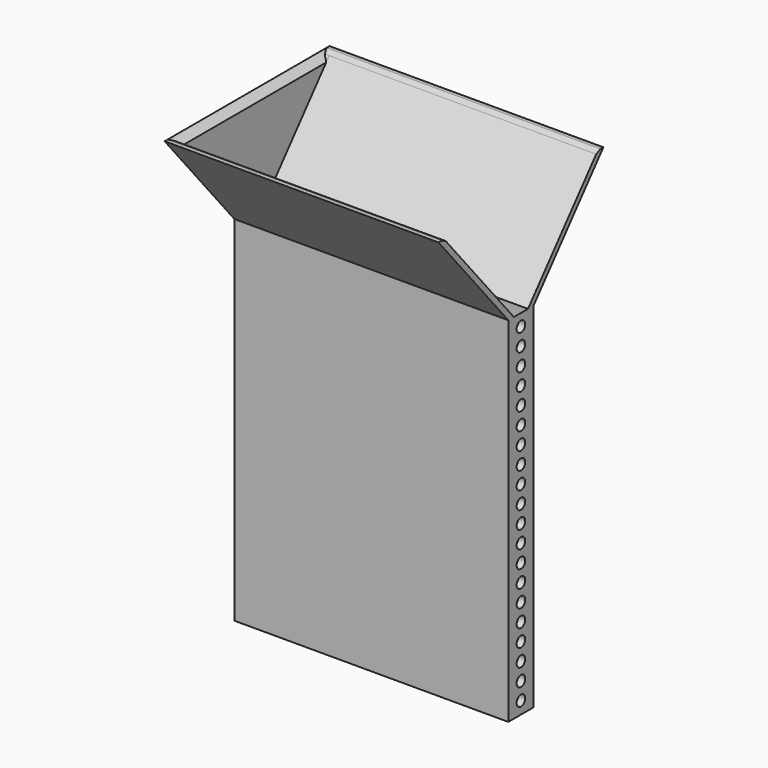
from build123d import *

# Parameters (mm, degrees)
F0_W         = 79
F0_H         = 9.1
F0_W_2       = 75
F0_H_2       = 5.1
F1_DEPTH     = 100
F0_W_3       = 55
F0_H_3       = 2.1
F2_DEPTH     = 2
F3_R         = 1.55
F4_DEPTH     = 79.001
F6_DEPTH     = 79
F7_DEPTH     = 2
F8_T1_DEPTH  = 5.1
F8_T3_DEPTH  = 79.5142210175
F8_T8_DEPTH  = 65.7327098225
F8_T15_DEPTH = 79.5142210175
F8_T20_DEPTH = 65.7327098225
F8_T28_DEPTH = 65.7327098225
F8_T33_DEPTH = 79.5142210175


# Not quite as in the source:
# - a fillet or chamfer that OpenCascade refuses, or shapes differently, is made with other operations: its cross-section is extruded or revolved along the edge and cut away or added


with BuildPart() as f1:
    # F0 (on Top) → F1 (new body)
    with BuildSketch(Plane.XY):
        Rectangle(F0_W, F0_H)
        Rectangle(F0_W_2, F0_H_2, mode=Mode.SUBTRACT)
    extrude(amount=F1_DEPTH)

    # F0 (on Top) → F2 (join)
    with BuildSketch(Plane.XY):
        Rectangle(F0_W, F0_H)
        Rectangle(F0_W_2, F0_H_2, mode=Mode.SUBTRACT)
        Rectangle(F0_W_2, F0_H_2)
        Rectangle(F0_W_3, F0_H_3, mode=Mode.SUBTRACT)
    extrude(amount=-F2_DEPTH)

    # F3 (on face) → F4 (cut, through all)
    with BuildSketch(Plane(origin=(-39.5, 0, 0), x_dir=(0, -1, 0), z_dir=(-1, 0, 0))):
        with BuildLine():
            ThreePointArc((0, 0), (1.0960155108, 0.4539844892), (1.55, 1.55))
            ThreePointArc((1.55, 1.55), (-1.0960155108, 2.6460155108), (0, 0))
        make_face()
        with Locations((0, 6.55)):
            Circle(F3_R)
        with Locations((0, 11.55)):
            Circle(F3_R)
        with Locations((0, 16.55)):
            Circle(F3_R)
        with Locations((0, 21.55)):
            Circle(F3_R)
        with Locations((0, 26.55)):
            Circle(F3_R)
        with Locations((0, 31.55)):
            Circle(F3_R)
        with Locations((0, 36.55)):
            Circle(F3_R)
        with Locations((0, 41.55)):
            Circle(F3_R)
        with Locations((0, 46.55)):
            Circle(F3_R)
        with Locations((0, 51.55)):
            Circle(F3_R)
        with Locations((0, 56.55)):
            Circle(F3_R)
        with Locations((0, 61.55)):
            Circle(F3_R)
        with Locations((0, 66.55)):
            Circle(F3_R)
        with Locations((0, 71.55)):
            Circle(F3_R)
        with Locations((0, 76.55)):
            Circle(F3_R)
        with Locations((0, 81.55)):
            Circle(F3_R)
        with Locations((0, 86.55)):
            Circle(F3_R)
        with Locations((0, 91.55)):
            Circle(F3_R)
        with Locations((0, 96.55)):
            Circle(F3_R)
    extrude(amount=-F4_DEPTH, mode=Mode.SUBTRACT)

    # F5 (on face) → F6 (join, through all)
    with BuildSketch(Plane(origin=(-39.5, 0, 0), x_dir=(0, -1, 0), z_dir=(-1, 0, 0))):
        Polygon((-29.7229889353, 130), (-4.55, 100), (-2.55, 100), (-27.7229889353, 130), align=None)
        Polygon((27.7229889353, 130), (2.55, 100), (4.55, 100), (29.7229889353, 130), align=None)
    extrude(amount=-F6_DEPTH)

    # F5 (on face) → F7 (join, through all)
    with BuildSketch(Plane(origin=(-39.5, 0, 0), x_dir=(0, -1, 0), z_dir=(-1, 0, 0))):
        Polygon((-27.7229889353, 130), (-2.55, 100), (2.55, 100), (27.7229889353, 130), align=None)
    extrude(amount=-F7_DEPTH)

    # F8: chamfer of 2 on 4 edges, made by hand

    # F8_s2 → F8_t1 (cut)
    with BuildSketch(Plane.XZ.offset(-2.55)):
        Polygon((37.5, 98), (39.5, 100), (37.5, 100), align=None)
    extrude(amount=F8_T1_DEPTH, mode=Mode.SUBTRACT)

    # F8_s4 → F8_t3 (cut)
    with BuildSketch(Plane.YZ.offset(-37.5)):
        Polygon((-28.6556042516, 130), (-27.1235153654, 129.2855752194), (-27.7229889353, 130), align=None)
        Polygon((28.6556042516, 130), (27.1235153654, 129.2855752194), (27.7229889353, 130), align=None)
    extrude(amount=F8_T3_DEPTH, mode=Mode.SUBTRACT)


with BuildPart() as f8_tool6:
    # F8_s7 → F8_t8 (new body)
    with BuildSketch(Plane.XZ.offset(32.8663549113)):
        Polygon((-39.5, 130), (-37.5, 128), (-37.5, 130), align=None)
    extrude(amount=-F8_T8_DEPTH)

    split(bisect_by=Plane(origin=(0, -47.7439862241, 40.0619612316), x_dir=(1, 0, 0), z_dir=(0, -0.7660444431, 0.6427876097)), keep=Keep.TOP)

    split(bisect_by=Plane(origin=(0, 47.7439862241, 40.0619612316), x_dir=(1, 0, 0), z_dir=(0, 0.7660444431, 0.6427876097)), keep=Keep.TOP)


with BuildPart() as f1_1:
    add(f1.part)

    # F8_t5: cut F8_tool6
    add(f8_tool6.part, mode=Mode.SUBTRACT)


with BuildPart() as f8_tool13:
    # F8_s14 → F8_t15 (new body)
    with BuildSketch(Plane.YZ.offset(-40.0142210175)):
        Polygon((-28.6556042516, 130), (-27.1235153654, 129.2855752194), (-27.7229889353, 130), align=None)
    extrude(amount=F8_T15_DEPTH)

    split(bisect_by=Plane.YZ.offset(-37.5), keep=Keep.BOTTOM)

    split(bisect_by=Plane.YZ.offset(-39.5), keep=Keep.TOP)


with BuildPart() as f8_tool18:
    # F8_s19 → F8_t20 (new body)
    with BuildSketch(Plane.XZ.offset(32.8663549113)):
        Polygon((-39.5, 130), (-37.5, 128), (-37.5, 130), align=None)
    extrude(amount=-F8_T20_DEPTH)

    split(bisect_by=Plane(origin=(0, 46.5703380464, 39.0771534786), x_dir=(1, 0, 0), z_dir=(0, 0.7660444431, 0.6427876097)), keep=Keep.TOP)

    split(bisect_by=Plane(origin=(0, 47.7439862241, 40.0619612316), x_dir=(1, 0, 0), z_dir=(0, -0.7660444431, -0.6427876097)), keep=Keep.TOP)


with BuildPart() as f8_tool13_1:
    add(f8_tool13.part)

    # F8_t23: intersect F8_tool18
    add(f8_tool18.part, mode=Mode.INTERSECT)


with BuildPart() as f1_2:
    add(f1_1.part)

    # F8_t11: cut F8_tool13
    add(f8_tool13_1.part, mode=Mode.SUBTRACT)


with BuildPart() as f8_tool26:
    # F8_s27 → F8_t28 (new body)
    with BuildSketch(Plane.XZ.offset(32.8663549113)):
        Polygon((-39.5, 130), (-37.5, 128), (-37.5, 130), align=None)
    extrude(amount=-F8_T28_DEPTH)

    split(bisect_by=Plane(origin=(0, -47.7439862241, 40.0619612316), x_dir=(1, 0, 0), z_dir=(0, 0.7660444431, -0.6427876097)), keep=Keep.TOP)

    split(bisect_by=Plane(origin=(0, -46.5703380464, 39.0771534786), x_dir=(1, 0, 0), z_dir=(0, -0.7660444431, 0.6427876097)), keep=Keep.TOP)


with BuildPart() as f8_tool31:
    # F8_s32 → F8_t33 (new body)
    with BuildSketch(Plane.YZ.offset(-40.0142210175)):
        Polygon((28.6556042516, 130), (27.1235153654, 129.2855752194), (27.7229889353, 130), align=None)
    extrude(amount=F8_T33_DEPTH)

    split(bisect_by=Plane.YZ.offset(-37.5), keep=Keep.BOTTOM)

    split(bisect_by=Plane.YZ.offset(-39.5), keep=Keep.TOP)


with BuildPart() as f8_tool26_1:
    add(f8_tool26.part)

    # F8_t36: intersect F8_tool31
    add(f8_tool31.part, mode=Mode.INTERSECT)


with BuildPart() as f1_3:
    add(f1_2.part)

    # F8_t24: cut F8_tool26
    add(f8_tool26_1.part, mode=Mode.SUBTRACT)


solid = f1_3.part
